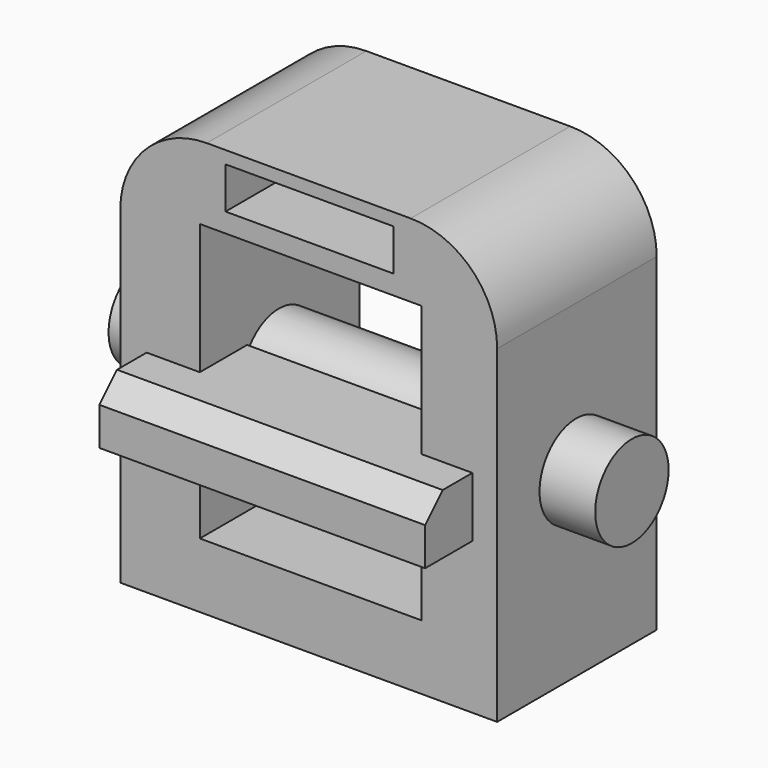
from build123d import *

# Parameters (mm, degrees)
F0_W      = 87.133936584
F0_H      = 95.9787741303
F1_DEPTH  = 46.1022332311
F2_W      = 51.2357354164
F2_H      = 64.0120953321
F3_DEPTH  = 79.969028011
F6_R      = 10.6062460881
F7_DEPTH  = 56.2525093555
F8_W      = 38.8421155512
F8_H      = 9.6180737019
F9_DEPTH  = 59.3906808645
F10_W     = 51.2357354164
F10_H     = 13.8573199511
F10_W_2   = 11.7768868804
F10_W_3   = 12.2887119651
F11_DEPTH = 13.6597724631
F12_R     = 20
F13_SIZE  = 5.08


# Not quite as in the source:
# - a feature names something its author has since deleted; it is built from what else it names
# - the program builds the solid bodies; features that only make, move or delete a surface that nothing else refers to are left out


with BuildPart() as f1:
    # F0 (on Front) → F1 (new body)
    with BuildSketch(Plane.XZ):
        with Locations((-0.1830421388, 6.0982592404)):
            Rectangle(F0_W, F0_H)
    extrude(amount=F1_DEPTH)

    # F2 (on face) → F3 (cut)
    with BuildSketch(Plane.XZ.offset(46.1022332311)):
        with Locations((0.2559125423, 5.0961896777)):
            Rectangle(F2_W, F2_H)
    extrude(amount=-F3_DEPTH, mode=Mode.SUBTRACT)

    # F6 (on Right) → F7 (join, symmetric)
    with BuildSketch(Plane.YZ):
        with Locations((-23.2529193163, 0)):
            Circle(F6_R)
    extrude(amount=F7_DEPTH, both=True)

    # F8 (on face) → F9 (cut)
    with BuildSketch(Plane(origin=(0, 0, 0), x_dir=(-1, 0, 0), z_dir=(0, 1, 0))):
        with Locations((0, 46.3703721762)):
            Rectangle(F8_W, F8_H)
    extrude(amount=-F9_DEPTH, mode=Mode.SUBTRACT)

    # F10 (on face) → F11 (join, symmetric)
    with BuildSketch(Plane.XZ.offset(46.1022332311)):
        with Locations((0.2559125423, 0)):
            Rectangle(F10_W, F10_H)
        with Locations((31.7622236907, 0)):
            Rectangle(F10_W_2, F10_H)
        with Locations((-31.5063111484, 0)):
            Rectangle(F10_W_3, F10_H)
    extrude(amount=F11_DEPTH, both=True)

    # F12
    f12_edges = [f1.edges().sort_by_distance(p)[0] for p in [
        (-43.75001, -23.051117, 54.087646),
        (43.383926, -23.051117, 54.087646),
    ]]
    fillet(f12_edges, radius=F12_R)

    # F13
    f13_edges = [f1.edges().sort_by_distance(p)[0] for p in [
        (0, -59.762006, 6.92866),
    ]]
    chamfer(f13_edges, length=F13_SIZE)


solid = f1.part
